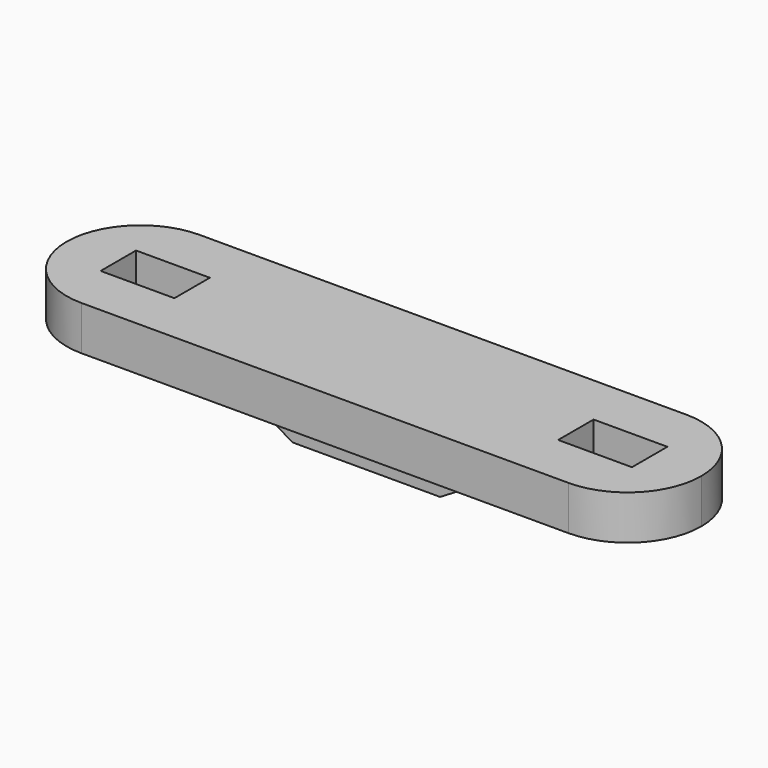
from build123d import *

# Parameters (mm, degrees)
F0_W       = 5
F0_H       = 3
F0_W_2     = 20
F1_DEPTH   = 3
F2_DEPTH   = 3
F3_SIZE2   = 4.99999
F3_SIZE    = 2.99999
F3_2_SIZE2 = 4.99999
F3_2_SIZE  = 2.99999


# Not quite as in the source:
# - a fillet or chamfer is up to 0.001 mm smaller than in the source, because OpenCascade refuses the exact size


with BuildPart() as f1:
    # F0 (on Top) → F1 (new body)
    with BuildSketch(Plane.XY):
        with BuildLine():
            Line((16.5, 10), (-16.5, 10))
            ThreePointArc((-16.5, 10), (-20.0355339059, 8.5355339059), (-21.5, 5))
            ThreePointArc((-21.5, 5), (-20.0355339059, 1.4644660941), (-16.5, 0))
            Line((-16.5, 0), (16.5, 0))
            ThreePointArc((16.5, 0), (20.0355339059, 1.4644660941), (21.5, 5))
            ThreePointArc((21.5, 5), (20.0355339059, 8.5355339059), (16.5, 10))
        make_face()
        with Locations((-15.5, 5)):
            Rectangle(F0_W, F0_H, mode=Mode.SUBTRACT)
        with Locations((0, 5)):
            Rectangle(F0_W_2, F0_H, mode=Mode.SUBTRACT)
        with Locations((15.5, 5)):
            Rectangle(F0_W, F0_H, mode=Mode.SUBTRACT)
        with Locations((0, 5)):
            Rectangle(F0_W_2, F0_H)
    extrude(amount=F1_DEPTH)

    # F0 (on Top) → F2 (join)
    with BuildSketch(Plane.XY):
        with Locations((0, 5)):
            Rectangle(F0_W_2, F0_H)
    extrude(amount=-F2_DEPTH)

    # F3 (size 3 and 5 in the source; OpenCascade refuses exactly that, so slightly less here)
    f3_edges = [f1.edges().sort_by_distance(p)[0] for p in [
        (-10, 5, -3),
    ]]
    f3_side = f1.faces().sort_by_distance((-10, 5, -1.5))[0]
    chamfer(f3_edges, length=F3_SIZE, length2=F3_SIZE2, reference=f3_side)

    # F3#2 (size 3 and 5 in the source; OpenCascade refuses exactly that, so slightly less here)
    f3_2_edges = [f1.edges().sort_by_distance(p)[0] for p in [
        (10, 5, -3),
    ]]
    f3_2_side = f1.faces().sort_by_distance((10, 5, -1.5))[0]
    chamfer(f3_2_edges, length=F3_2_SIZE, length2=F3_2_SIZE2, reference=f3_2_side)


solid = f1.part
